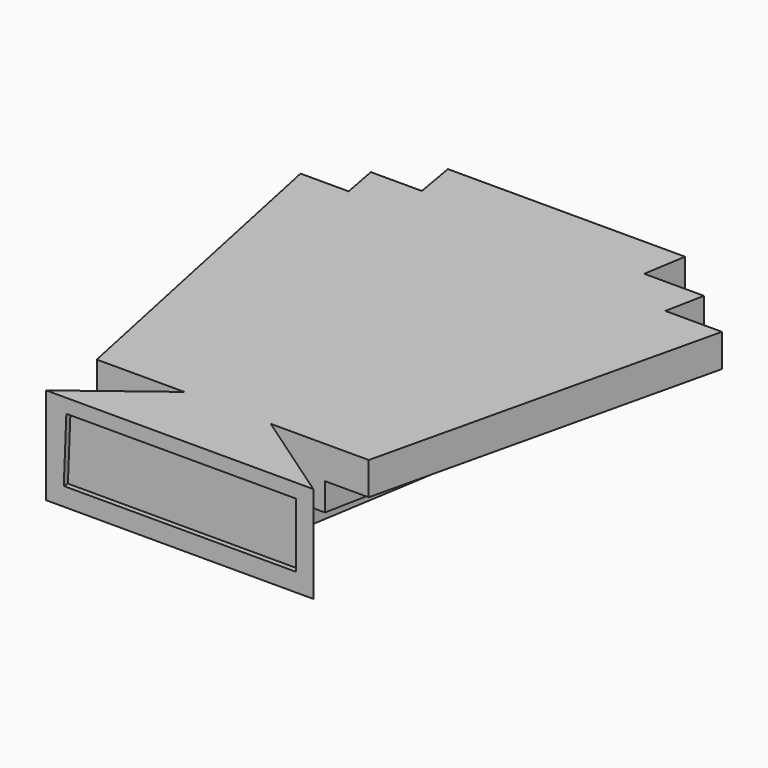
from build123d import *

# Parameters (mm, degrees)
F1_DEPTH      = 14.478
F3_DEPTH      = 9.906
F5_DEPTH      = 8.89
F7_DEPTH      = 5.334
F9_DEPTH      = 4.826
F11_DEPTH     = 12.7
F13_DEPTH     = 0.254
F15_DEPTH     = 0.4318
F17_DEPTH     = 0.254
F19_DEPTH     = 0.4572
F21_DEPTH     = 0.4318
F23_DEPTH     = 0.635
F25_DEPTH     = 14.224
F27_DEPTH     = 0.762
F29_DEPTH     = 0.762
F30_W         = 6.4463028684
F30_H         = 5.498317536
F31_DEPTH     = 0.508
F32_W         = 8.5394121706
F32_H         = 5.5236583576
F34_DEPTH     = 0.889
F35_DEPTH     = 0.9652
F36_TEXT_SIZE = 6.9039058872
F37_DEPTH     = 0.6096
F38_TEXT_SIZE = 6.0501663635
F39_DEPTH     = 0.508


# Not quite as in the source:
# - Text() gives the source's letters only with a copy of the font that has no kerning and outlines rounded to 1/6400 em; it was checked with that copy


with BuildPart() as f1:
    # F0 (on Top) → F1 (new body)
    with BuildSketch(Plane.XY):
        Polygon((17.9169289768, 22.2776643932), (-16.9689450413, 22.2776643932), (-6.1619086191, -39.9102047086), (7.8682815656, -39.9102047086), align=None)
    extrude(amount=F1_DEPTH)

    # F2 (on face) → F3 (join)
    with BuildSketch(Plane.XY.offset(14.478)):
        Polygon((-6.1619086191, -39.9102047086), (-15.9066021967, 16.164532617), (-23.415248841, 16.164532617), (-12.7978082746, -39.9102047086), align=None)
    extrude(amount=-F3_DEPTH)

    # F4 (on face) → F5 (join)
    with BuildSketch(Plane.XY.offset(14.478)):
        Polygon((25.6904140115, 16.0308813217), (16.9075404667, 16.0308813217), (7.8682815656, -39.9102047086), (14.6937789395, -39.9102047086), align=None)
    extrude(amount=-F5_DEPTH)

    # F6 (on face) → F7 (join)
    with BuildSketch(Plane.XY.offset(14.478)):
        Polygon((-12.7978082746, -39.9102047086), (-22.4054939063, 10.8316331883), (-29.4823590666, 10.8316331883), (-18.8649166375, -39.9102047086), align=None)
    extrude(amount=-F7_DEPTH)

    # F8 (on face) → F9 (join)
    with BuildSketch(Plane.XY.offset(14.478)):
        Polygon((32.8951068223, 10.329728196), (24.5697081965, 10.329728196), (14.6937789395, -39.9102047086), (21.1400836706, -39.9102047086), align=None)
    extrude(amount=-F9_DEPTH)

    # F10 (on face) → F11 (cut)
    with BuildSketch(Plane(origin=(0, 0, 0), x_dir=(1, 0, 0), z_dir=(0, 0, -1))):
        Polygon((-12.8096845001, -18.7246967107), (13.0148036405, -18.7246967107), (4.7607147135, 34.3760251999), (-4.2147650383, 34.3760251999), align=None)
    extrude(amount=-F11_DEPTH, mode=Mode.SUBTRACT)

    # F12 (on face) → F13 (join)
    with BuildSketch(Plane(origin=(0, 0, 0), x_dir=(1, 0, 0), z_dir=(0, 0, -1))):
        Polygon((-12.8096845001, -18.7246967107), (12.1590542954, -13.2194364207), (11.566128713, -9.4049904236), (-12.1385823924, -14.5785256436), align=None)
    extrude(amount=-F13_DEPTH)

    # F14 (on face) → F15 (join)
    with BuildSketch(Plane(origin=(0, 0, 0), x_dir=(1, 0, 0), z_dir=(0, 0, -1))):
        Polygon((-11.4159222756, -10.1138213415), (10.8921530542, -5.0691279989), (10.2214565149, -0.7543610106), (-10.6257552963, -5.2320493576), align=None)
    extrude(amount=-F15_DEPTH)

    # F16 (on face) → F17 (join)
    with BuildSketch(Plane(origin=(0, 0, 0), x_dir=(1, 0, 0), z_dir=(0, 0, -1))):
        Polygon((-9.9267917791, -0.9137462581), (9.574702169, 3.4063795597), (8.9401933703, 7.4883413077), (-9.1725084385, 3.7463311387), align=None)
    extrude(amount=-F17_DEPTH)

    # F18 (on face) → F19 (join)
    with BuildSketch(Plane(origin=(0, 0, 0), x_dir=(1, 0, 0), z_dir=(0, 0, -1))):
        Polygon((-8.4142207972, 8.4311477153), (8.2788480639, 11.7429493589), (7.8372463907, 14.5838889043), (-7.8120701883, 12.1513259175), align=None)
    extrude(amount=-F19_DEPTH)

    # F20 (on face) → F21 (join)
    with BuildSketch(Plane(origin=(0, 0, 0), x_dir=(1, 0, 0), z_dir=(0, 0, -1))):
        Polygon((-7.0233491057, 17.0241649312), (7.1162794167, 19.222058802), (6.6450210951, 22.2537873554), (-6.5078034746, 20.2092843857), align=None)
    extrude(amount=-F21_DEPTH)

    # F22 (on face) → F23 (join)
    with BuildSketch(Plane(origin=(0, 0, 0), x_dir=(1, 0, 0), z_dir=(0, 0, -1))):
        Polygon((-5.8580149442, 24.2237769248), (5.9609496436, 26.6545986666), (5.4314066052, 30.0612881106), (-5.1801374805, 28.4118071735), align=None)
    extrude(amount=-F23_DEPTH)

    # F24 (on face) → F25 (join)
    with BuildSketch(Plane.XY.offset(14.478)):
        Polygon((6.7307003774, -39.9102047086), (-5.9723109007, -39.9102047086), (-18.6222587873, -49.5328344405), (20.6796713173, -49.5328344405), align=None)
    extrude(amount=-F25_DEPTH)

    # F26 (on face) → F27 (cut)
    with BuildSketch(Plane.XZ.offset(49.5328344405)):
        Polygon((18.1065294892, 12.4186137691), (-15.641765669, 12.4186137691), (-16.0209592432, 2.9387560207), (18.1065294892, 2.9387560207), align=None)
    extrude(amount=-F27_DEPTH, mode=Mode.SUBTRACT)

    # F28 (on face) → F29 (join)
    with BuildSketch(Plane(origin=(0, 22.2776643932, 0), x_dir=(-1, 0, 0), z_dir=(0, 1, 0))):
        Polygon((-1.3013028074, 9.5394384116), (-5.8367066085, 9.5394384116), (-5.9723113663, 4.0763388388), (-1.3013028074, 4.0763388388), align=None)
    extrude(amount=F29_DEPTH)

    # F30 (on face) → F31 (join)
    with BuildSketch(Plane(origin=(0, 22.2776643932, 0), x_dir=(-1, 0, 0), z_dir=(0, 1, 0))):
        with Locations((11.470626574, 6.8254976068)):
            Rectangle(F30_W, F30_H)
    extrude(amount=F31_DEPTH)

    # F32 (on face) → F34 (join)
    with BuildSketch(Plane(origin=(0, 22.2776643932, 0), x_dir=(-1, 0, 0), z_dir=(0, 1, 0))):
        with Locations((-12.4385040253, 10.7616805471)):
            Rectangle(F32_W, F32_H)
    extrude(amount=F34_DEPTH)

    # F33 (on face) → F35 (join)
    with BuildSketch(Plane(origin=(0, 22.2776643932, 0), x_dir=(-1, 0, 0), z_dir=(0, 1, 0))):
        Polygon((-8.1682298332, 8.0320574343), (-8.16879794, 8.0320574343), (-8.16879794, 7.9998513684), (-16.6673008353, 7.9998513684), (-16.6673008353, 2.6109684259), (-8.1682298332, 2.6109684259), align=None)
    extrude(amount=F35_DEPTH)

    # F36 (on face) → F37 (join)
    with BuildSketch(Plane(origin=(0, 23.1666643932, 0), x_dir=(-1, 0, 0), z_dir=(0, 1, 0))):
        with Locations((-14.5036997274, 7.9998513684)):
            Text('+', F36_TEXT_SIZE, font='Open Sans', font_style=FontStyle.BOLD, text_align=(TextAlign.LEFT, TextAlign.BOTTOM))
    extrude(amount=F37_DEPTH)

    # F38 (on face) → F39 (join)
    with BuildSketch(Plane(origin=(0, 23.2428643932, 0), x_dir=(-1, 0, 0), z_dir=(0, 1, 0))):
        with Locations((-13.4615572169, 3.8313609548)):
            Text('-', F38_TEXT_SIZE, font='Open Sans', font_style=FontStyle.BOLD, text_align=(TextAlign.LEFT, TextAlign.BOTTOM))
    extrude(amount=F39_DEPTH)


solid = f1.part
